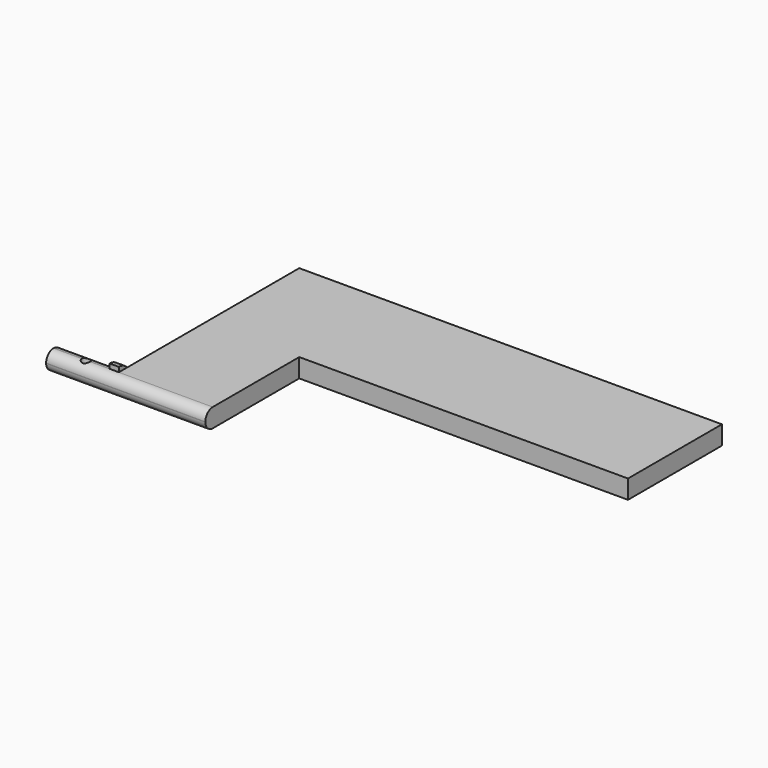
from build123d import *

# Parameters (mm, degrees)
F0_W        = 17.6611579955
F0_H        = 5.08
F1_DEPTH    = 5.08
F2_T1_DEPTH = 55.76598658
F2_T3_DEPTH = 24.0135722877
F4_DEPTH    = 5.081
F6_DEPTH    = 2.54


# Not quite as in the source:
# - a fillet or chamfer that OpenCascade refuses, or shapes differently, is made with other operations: its cross-section is extruded or revolved along the edge and cut away or added


with BuildPart() as f1:
    # F0 (on Top) → F1 (new body)
    with BuildSketch(Plane.XY):
        with Locations((-8.8305789977, 2.54)):
            Rectangle(F0_W, F0_H)
        Polygon((0, 5.08), (0, 0), (25.4, 0), (25.4, 31.75), (88.9, 31.75), (114.3, 31.75), (114.3, 63.5), (0, 63.5), (0, 28.7528), align=None)
    extrude(amount=F1_DEPTH)

    # F2: fillet of radius 2.54 on 4 edges, made by hand

    # F2_s2 → F2_t1 (cut)
    with BuildSketch(Plane.YZ.offset(-24.0135722877)):
        with BuildLine():
            ThreePointArc((-0.0004, 2.5390343146), (0.7439487758, 4.3360512242), (2.5409656854, 5.0804))
            Line((2.5409656854, 5.0804), (2.5409656854, 5.3345365685))
            ThreePointArc((2.5409656854, 5.3345365685), (1.2704828427, 5.3341365685), (0, 5.3341365685))
            Line((0, 5.3341365685), (-0.2541365685, 5.08))
            ThreePointArc((-0.2541365685, 5.08), (-0.2541365685, 3.8095171573), (-0.2545365685, 2.5390343146))
            Line((-0.2545365685, 2.5390343146), (-0.0004, 2.5390343146))
        make_face()
        with BuildLine():
            ThreePointArc((-0.0004, 2.5409656854), (0.7439487758, 0.7439487758), (2.5409656854, -0.0004))
            Line((2.5409656854, -0.0004), (2.5409656854, -0.2545365685))
            ThreePointArc((2.5409656854, -0.2545365685), (1.2704828427, -0.2541365685), (0, -0.2541365685))
            Line((0, -0.2541365685), (-0.2541365685, 0))
            ThreePointArc((-0.2541365685, 0), (-0.2541365685, 1.2704828427), (-0.2545365685, 2.5409656854))
            Line((-0.2545365685, 2.5409656854), (-0.0004, 2.5409656854))
        make_face()
    extrude(amount=F2_T1_DEPTH, mode=Mode.SUBTRACT)

    # F2_s4 → F2_t3 (cut)
    with BuildSketch(Plane.YZ.offset(-24.0135722877)):
        with BuildLine():
            ThreePointArc((5.0804, 2.5390343146), (4.3360512242, 4.3360512242), (2.5390343146, 5.0804))
            Line((2.5390343146, 5.0804), (2.5390343146, 5.3345365685))
            ThreePointArc((2.5390343146, 5.3345365685), (3.8095171573, 5.3341365685), (5.08, 5.3341365685))
            Line((5.08, 5.3341365685), (5.3341365685, 5.08))
            ThreePointArc((5.3341365685, 5.08), (5.3341365685, 3.8095171573), (5.3345365685, 2.5390343146))
            Line((5.3345365685, 2.5390343146), (5.0804, 2.5390343146))
        make_face()
        with BuildLine():
            ThreePointArc((5.0804, 2.5409656854), (4.3360512242, 0.7439487758), (2.5390343146, -0.0004))
            Line((2.5390343146, -0.0004), (2.5390343146, -0.2545365685))
            ThreePointArc((2.5390343146, -0.2545365685), (3.8095171573, -0.2541365685), (5.08, -0.2541365685))
            Line((5.08, -0.2541365685), (5.3341365685, 0))
            ThreePointArc((5.3341365685, 0), (5.3341365685, 1.2704828427), (5.3345365685, 2.5409656854))
            Line((5.3345365685, 2.5409656854), (5.0804, 2.5409656854))
        make_face()
    extrude(amount=F2_T3_DEPTH, mode=Mode.SUBTRACT)

    # F3 (on face) → F4 (cut, through all)
    with BuildSketch(Plane.XY.offset(5.08)):
        with BuildLine():
            ThreePointArc((-7.7692847717, 2.54), (-8.89, 3.6607152283), (-10.0107152283, 2.54))
            Line((-10.0107152283, 2.54), (-7.7692847717, 2.54))
        make_face()
        with BuildLine():
            Line((-7.7692847717, 2.54), (-10.0107152283, 2.54))
            ThreePointArc((-10.0107152283, 2.54), (-8.89, 1.4192847717), (-7.7692847717, 2.54))
        make_face()
    extrude(amount=-F4_DEPTH, mode=Mode.SUBTRACT)

    # F5 (on face) → F6 (join)
    with BuildSketch(Plane(origin=(0, 0, 0), x_dir=(0, -1, 0), z_dir=(-1, 0, 0))):
        with BuildLine():
            Line((-2.54, 2.54), (-2.54, 6.35))
            ThreePointArc((-2.54, 6.35), (-4.0954259867, 6.0180382402), (-5.3798063314, 5.08))
            Line((-5.3798063314, 5.08), (-2.5841223678, 5.08))
            ThreePointArc((-2.5841223678, 5.08), (-4.3360512242, 4.3360512242), (-5.08, 2.5841223678))
            Line((-5.08, 2.5841223678), (-5.08, 2.54))
            Line((-5.08, 2.54), (-2.54, 2.54))
        make_face()
        with BuildLine():
            ThreePointArc((-6.35, 2.54), (-6.0991966876, 1.180507838), (-5.3798063314, 0))
            Line((-5.3798063314, 0), (-2.5841223678, 0))
            ThreePointArc((-2.5841223678, 0), (-4.3360512242, 0.7439487758), (-5.08, 2.4958776322))
            Line((-5.08, 2.4958776322), (-5.08, 2.54))
            Line((-5.08, 2.54), (-6.35, 2.54))
        make_face()
        with BuildLine():
            Line((-2.5841223678, 5.08), (-5.3798063314, 5.08))
            ThreePointArc((-5.3798063314, 5.08), (-6.0991966876, 3.899492162), (-6.35, 2.54))
            Line((-6.35, 2.54), (-5.08, 2.54))
            Line((-5.08, 2.54), (-5.08, 2.5841223678))
            ThreePointArc((-5.08, 2.5841223678), (-4.3360512242, 4.3360512242), (-2.5841223678, 5.08))
        make_face()
        with BuildLine():
            Line((-2.54, 0), (-2.54, 2.54))
            Line((-2.54, 2.54), (-5.08, 2.54))
            Line((-5.08, 2.54), (-5.08, 2.4958776322))
            ThreePointArc((-5.08, 2.4958776322), (-4.3360512242, 0.7439487758), (-2.5841223678, 0))
            Line((-2.5841223678, 0), (-2.54, 0))
        make_face()
    extrude(amount=F6_DEPTH)


solid = f1.part
